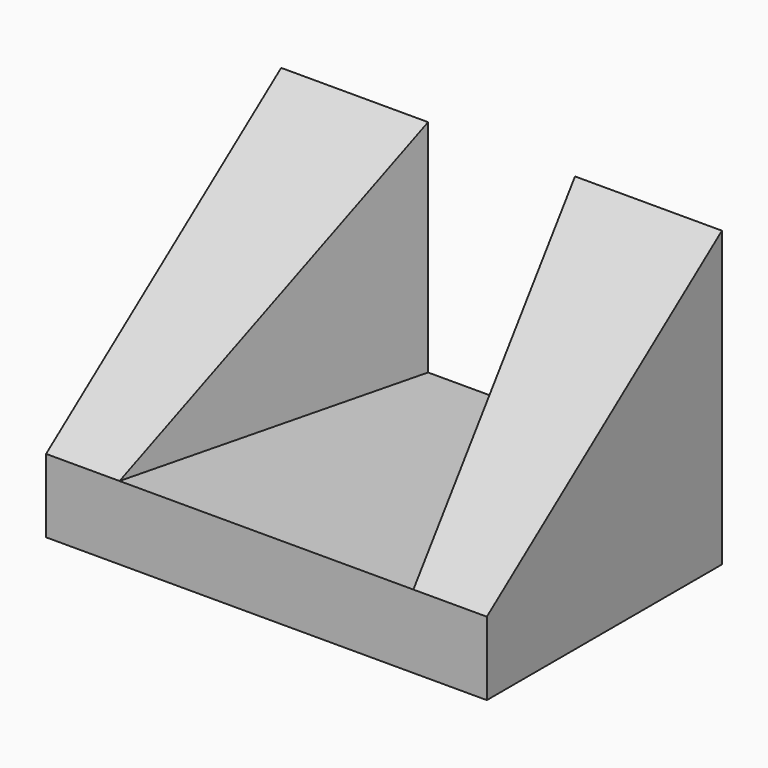
from build123d import *

# Parameters (mm, degrees)
F1_DEPTH   = 10
F2_DEPTH   = 30
F3_SIZE2   = 29.99999
F3_SIZE    = 39.99999
F3_2_SIZE2 = 29.99999
F3_2_SIZE  = 39.99999


# Not quite as in the source:
# - a fillet or chamfer is up to 0.001 mm smaller than in the source, because OpenCascade refuses the exact size


with BuildPart() as f1:
    # F0 (on Top) → F1 (new body)
    with BuildSketch(Plane.XY):
        Polygon((0, 40), (0, 0), (10, 0), (20, 40), align=None)
        Polygon((20, 40), (10, 0), (50, 0), (40, 40), align=None)
        Polygon((40, 40), (50, 0), (60, 0), (60, 40), align=None)
    extrude(amount=-F1_DEPTH)

    # F0 (on Top) → F2 (join)
    with BuildSketch(Plane.XY):
        Polygon((0, 40), (0, 0), (10, 0), (20, 40), align=None)
        Polygon((40, 40), (50, 0), (60, 0), (60, 40), align=None)
    extrude(amount=F2_DEPTH)

    # F3 (size 40 and 30 in the source; OpenCascade refuses exactly that, so slightly less here)
    f3_edges = [f1.edges().sort_by_distance(p)[0] for p in [
        (5, 0, 30),
    ]]
    f3_side = f1.faces().sort_by_distance((7.777778, 22.222222, 30))[0]
    chamfer(f3_edges, length=F3_SIZE, length2=F3_SIZE2, reference=f3_side)

    # F3#2 (size 40 and 30 in the source; OpenCascade refuses exactly that, so slightly less here)
    f3_2_edges = [f1.edges().sort_by_distance(p)[0] for p in [
        (55, 0, 30),
    ]]
    f3_2_side = f1.faces().sort_by_distance((52.222222, 22.222222, 30))[0]
    chamfer(f3_2_edges, length=F3_2_SIZE, length2=F3_2_SIZE2, reference=f3_2_side)


solid = f1.part
